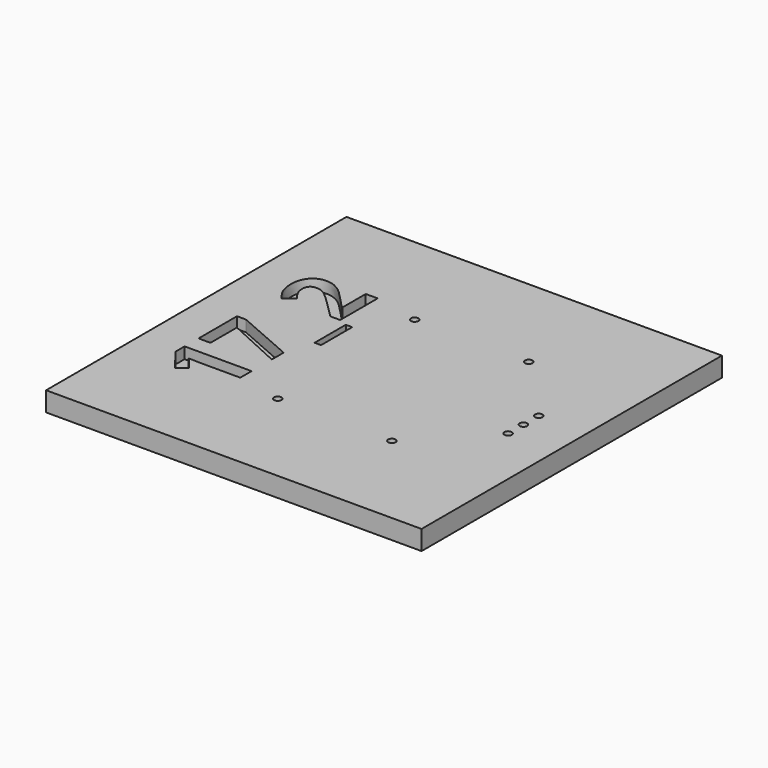
from build123d import *

# Parameters (mm, degrees)
F0_W         = 50
F0_H         = 50
F1_DEPTH     = 2.6
F2_TEXT_SIZE = 12.5
F3_DEPTH     = 1.5
F4_R         = 0.5
F5_DEPTH     = 2.6


# Not quite as in the source:
# - Text() gives the source's letters only with a copy of the font that has no kerning and outlines rounded to 1/6400 em; it was checked with that copy


with BuildPart() as f1:
    # F0 (on Top) → F1 (new body)
    with BuildSketch(Plane.XY):
        with Locations((-18.1587231159, 3.3350909071)):
            Rectangle(F0_W, F0_H)
    extrude(amount=F1_DEPTH)

    # F2 (on face) → F3 (cut)
    with BuildSketch(Plane.XY.offset(2.6)):
        with Locations(Location((-29.1587231159, -10.1149090929), (0, 0, 90))):
            Text('17_2', F2_TEXT_SIZE, font='Open Sans', font_style=FontStyle.BOLD, text_align=(TextAlign.LEFT, TextAlign.BOTTOM))
    extrude(amount=-F3_DEPTH, mode=Mode.SUBTRACT)

    # F4 (on face) → F5 (cut, through all)
    with BuildSketch(Plane.XY.offset(2.6)):
        with Locations((-23.1587231159, -8.1049090929)):
            Circle(F4_R)
        with Locations((-23.1587231159, 14.6950909071)):
            Circle(F4_R)
        with Locations((-7.9587231159, -8.1049090929)):
            Circle(F4_R)
        with Locations((-7.9587231159, 14.6950909071)):
            Circle(F4_R)
        with Locations((0.4412768841, 0.7550909071)):
            Circle(F4_R)
        with Locations((0.4412768841, 3.2950909071)):
            Circle(F4_R)
        with Locations((0.4412768841, 5.8350909071)):
            Circle(F4_R)
    extrude(amount=-F5_DEPTH, mode=Mode.SUBTRACT)


solid = f1.part
